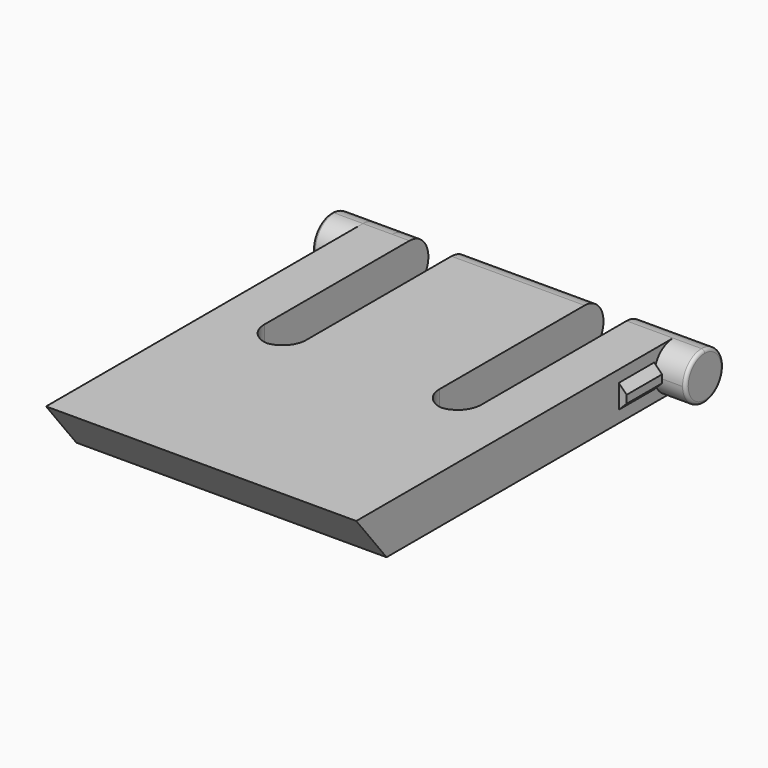
from build123d import *

# Parameters (mm, degrees)
F1_DEPTH      = 3
F3_DEPTH      = 2
F5_DEPTH      = 2
F6_DEPTH      = 0.5
F7_SIZE       = 0.49999
F8_DEPTH      = 0.5
F9_SIZE       = 0.49999
F10_DEPTH     = 19.66
F11_R         = 1.4999
F12_T3_DEPTH  = 3
F12_T6_DEPTH  = 3
F12_T9_DEPTH  = 3
F12_T12_DEPTH = 3
F12_T16_DEPTH = 15.94
F12_T19_DEPTH = 10.45
F12_T22_DEPTH = 15.94
F12_T25_DEPTH = 10.45
F14_T3_ANGLE  = 179.9999999988
F14_T6_ANGLE  = 90
F14_T9_ANGLE  = 90.0000000012


# Not quite as in the source:
# - a fillet or chamfer that OpenCascade refuses, or shapes differently, is made with other operations: its cross-section is extruded or revolved along the edge and cut away or added
# - two fillets or chamfers of one size are made in one step
# - a fillet or chamfer is up to 0.001 mm smaller than in the source, because OpenCascade refuses the exact size


with BuildPart() as f1:
    # F0 (on Top) → F1 (new body)
    with BuildSketch(Plane.XY):
        Polygon((-26.8430960169, 15.6478737652), (-29.7930960169, 15.6478737652), (-29.7930960169, -10.9521262348), (-10.1330960169, -10.9521262348), (-10.1330960169, 15.6478737652), (-13.0830960169, 15.6478737652), (-13.0830960169, 1.1478737652), (-15.7430960169, 1.1478737652), (-15.7430960169, 15.6478737652), (-24.1830960169, 15.6478737652), (-24.1830960169, 1.1478737652), (-26.8430960169, 1.1478737652), align=None)
    extrude(amount=F1_DEPTH)

    # F2 (on face) → F3 (join)
    with BuildSketch(Plane.YZ.offset(-10.1330960169)):
        with BuildLine():
            ThreePointArc((14.1478737652, 0), (15.208533937, 0.4393398282), (15.6478737652, 1.5))
            ThreePointArc((15.6478737652, 1.5), (15.208533937, 2.5606601718), (14.1478737652, 3))
            ThreePointArc((14.1478737652, 3), (13.0872135935, 2.5606601718), (12.6478737652, 1.5))
            ThreePointArc((12.6478737652, 1.5), (13.0872135935, 0.4393398282), (14.1478737652, 0))
        make_face()
    extrude(amount=F3_DEPTH)

    # F4 (on face) → F5 (join)
    with BuildSketch(Plane(origin=(-29.7930960169, 0, 0), x_dir=(0, -1, 0), z_dir=(-1, 0, 0))):
        with BuildLine():
            ThreePointArc((-14.1478737652, 0), (-13.0872135935, 0.4393398282), (-12.6478737652, 1.5))
            ThreePointArc((-12.6478737652, 1.5), (-13.0872135935, 2.5606601718), (-14.1478737652, 3))
            ThreePointArc((-14.1478737652, 3), (-15.2085339334, 2.5606601754), (-15.6478737652, 1.5000000103))
            ThreePointArc((-15.6478737652, 1.5000000103), (-15.2085339407, 0.4393398319), (-14.1478737652, 0))
        make_face()
    extrude(amount=F5_DEPTH)

    # F4 (on face) → F10 (cut, through all)
    with BuildSketch(Plane(origin=(-29.7930960169, 0, 0), x_dir=(0, -1, 0), z_dir=(-1, 0, 0))):
        Polygon((10.9521262348, 0), (10.9521262348, 3), (8.5521262348, 0), align=None)
    extrude(amount=-F10_DEPTH, mode=Mode.SUBTRACT)

    # F11 (radius 1.5 in the source; OpenCascade refuses exactly that, so slightly less here)
    f11_edges = [f1.edges().sort_by_distance(p)[0] for p in [
        (-28.318096, 15.647874, 3),
        (-28.318096, 15.647874, 0),
    ]]
    fillet(f11_edges, radius=F11_R)

    # F12: fillet of radius 1.5 on 8 edges, made by hand


with BuildPart() as f6:
    # F4 (on face) → F6 (new body)
    with BuildSketch(Plane(origin=(-29.7930960169, 0, 0), x_dir=(0, -1, 0), z_dir=(-1, 0, 0))):
        Polygon((-12.6478737652, 2.25), (-12.6478737652, 1.5), (-12.6478737652, 0.75), (-9.8478737652, 0.75), (-9.8478737652, 1.5), (-9.8478737652, 2.25), align=None)
    extrude(amount=F6_DEPTH)

    # F7 (size 0.5 in the source; OpenCascade refuses exactly that, so slightly less here)
    f7_edges = [f6.edges().sort_by_distance(p)[0] for p in [
        (-30.293096, 11.247874, 0.75),
        (-30.293096, 11.247874, 2.25),
    ]]
    chamfer(f7_edges, length=F7_SIZE)


with BuildPart() as f8:
    # F2 (on face) → F8 (new body)
    with BuildSketch(Plane.YZ.offset(-10.1330960169)):
        Polygon((12.6478737652, 0.75), (12.6478737652, 1.5), (12.6478737652, 2.25), (9.8478737652, 2.25), (9.8478737652, 0.75), align=None)
    extrude(amount=F8_DEPTH)

    # F9 (size 0.5 in the source; OpenCascade refuses exactly that, so slightly less here)
    f9_edges = [f8.edges().sort_by_distance(p)[0] for p in [
        (-9.633096, 11.247874, 2.25),
        (-9.633096, 11.247874, 0.75),
    ]]
    chamfer(f9_edges, length=F9_SIZE)


with BuildPart() as f12_tool1:
    # F12_s2 → F12_t3 (new body)
    with BuildSketch(Plane.XY):
        with BuildLine():
            ThreePointArc((-26.8430960169, 2.6478737652), (-26.4037561887, 1.5872135935), (-25.3430960169, 1.1478737652))
            Line((-25.3430960169, 1.1478737652), (-26.8430960169, 1.1478737652))
            Line((-26.8430960169, 1.1478737652), (-26.8430960169, 2.6478737652))
        make_face()
    extrude(amount=F12_T3_DEPTH)


with BuildPart() as f12_tool4:
    # F12_s5 → F12_t6 (new body)
    with BuildSketch(Plane.XY):
        with BuildLine():
            ThreePointArc((-25.6830960169, 1.1478737652), (-24.6224358452, 1.5872135935), (-24.1830960169, 2.6478737652))
            Line((-24.1830960169, 2.6478737652), (-24.1830960169, 1.1478737652))
            Line((-24.1830960169, 1.1478737652), (-25.6830960169, 1.1478737652))
        make_face()
    extrude(amount=F12_T6_DEPTH)


with BuildPart() as f12_tool7:
    # F12_s8 → F12_t9 (new body)
    with BuildSketch(Plane.XY):
        with BuildLine():
            ThreePointArc((-15.7430960169, 2.6478737652), (-15.3037561887, 1.5872135935), (-14.2430960169, 1.1478737652))
            Line((-14.2430960169, 1.1478737652), (-15.7430960169, 1.1478737652))
            Line((-15.7430960169, 1.1478737652), (-15.7430960169, 2.6478737652))
        make_face()
    extrude(amount=F12_T9_DEPTH)


with BuildPart() as f12_tool10:
    # F12_s11 → F12_t12 (new body)
    with BuildSketch(Plane.XY):
        with BuildLine():
            ThreePointArc((-13.0830960169, 2.6478737652), (-13.5224358452, 1.5872135935), (-14.5830960169, 1.1478737652))
            Line((-14.5830960169, 1.1478737652), (-13.0830960169, 1.1478737652))
            Line((-13.0830960169, 1.1478737652), (-13.0830960169, 2.6478737652))
        make_face()
    extrude(amount=F12_T12_DEPTH)


with BuildPart() as f1_1:
    add(f1.part)

    # F12_t13: union F12_tool1, F12_tool4, F12_tool7, F12_tool10
    add([f12_tool1.part, f12_tool4.part, f12_tool7.part, f12_tool10.part])


with BuildPart() as f12_tool14:
    # F12_s15 → F12_t16 (new body)
    with BuildSketch(Plane.YZ.offset(-11.9930960169)):
        with BuildLine():
            ThreePointArc((14.1478737652, 0), (15.208533937, 0.4393398282), (15.6478737652, 1.5))
            Line((15.6478737652, 1.5), (15.6478737652, 0))
            Line((15.6478737652, 0), (14.1478737652, 0))
        make_face()
    extrude(amount=-F12_T16_DEPTH)


with BuildPart() as f12_tool17:
    # F12_s18 → F12_t19 (new body)
    with BuildSketch(Plane.YZ.offset(-6.3830960169)):
        with BuildLine():
            ThreePointArc((14.1478737652, 0), (15.208533937, 0.4393398282), (15.6478737652, 1.5))
            Line((15.6478737652, 1.5), (15.6478737652, 0))
            Line((15.6478737652, 0), (14.1478737652, 0))
        make_face()
    extrude(amount=-F12_T19_DEPTH)


with BuildPart() as f12_tool20:
    # F12_s21 → F12_t22 (new body)
    with BuildSketch(Plane.YZ.offset(-11.9930960169)):
        with BuildLine():
            ThreePointArc((15.6478737652, 1.5), (15.208533937, 2.5606601718), (14.1478737652, 3))
            Line((14.1478737652, 3), (15.6478737652, 3))
            Line((15.6478737652, 3), (15.6478737652, 1.5))
        make_face()
    extrude(amount=-F12_T22_DEPTH)


with BuildPart() as f12_tool23:
    # F12_s24 → F12_t25 (new body)
    with BuildSketch(Plane.YZ.offset(-6.3830960169)):
        with BuildLine():
            ThreePointArc((15.6478737652, 1.5), (15.208533937, 2.5606601718), (14.1478737652, 3))
            Line((14.1478737652, 3), (15.6478737652, 3))
            Line((15.6478737652, 3), (15.6478737652, 1.5))
        make_face()
    extrude(amount=-F12_T25_DEPTH)


with BuildPart() as f1_2:
    add(f1_1.part)

    # F12_t26: cut F12_tool14, F12_tool17, F12_tool20, F12_tool23
    add([f12_tool14.part, f12_tool17.part, f12_tool20.part, f12_tool23.part], mode=Mode.SUBTRACT)

    # F14: fillet of radius 0.2 on 1 edges, made by hand


with BuildPart() as f14_tool1:
    # F14_s2 → F14_t3 (revolve)
    with BuildSketch(Plane.XZ.offset(-14.1478737652)):
        with BuildLine():
            ThreePointArc((-8.1330960169, 0.2), (-8.1916746607, 0.0585786438), (-8.3330960169, 0))
            Line((-8.3330960169, 0), (-8.1330960169, 0))
            Line((-8.1330960169, 0), (-8.1330960169, 0.2))
        make_face()
    revolve(axis=Axis((-8.1330960169, 14.1478737652, 1.5), (-1, 0, 0)), revolution_arc=F14_T3_ANGLE)


with BuildPart() as f14_tool4:
    # F14_s5 → F14_t6 (revolve)
    with BuildSketch(Plane.XY.offset(1.5)):
        with BuildLine():
            ThreePointArc((-8.3330960169, 15.6478737652), (-8.1916746607, 15.5892951215), (-8.1330960169, 15.4478737652))
            Line((-8.1330960169, 15.4478737652), (-8.1330960169, 15.6478737652))
            Line((-8.1330960169, 15.6478737652), (-8.3330960169, 15.6478737652))
        make_face()
    revolve(axis=Axis((-8.1330960169, 14.1478737652, 1.5), (-1, 0, 0)), revolution_arc=F14_T6_ANGLE)


with BuildPart() as f14_tool7:
    # F14_s8 → F14_t9 (revolve)
    with BuildSketch(Plane.XZ.offset(-14.1478737652)):
        with BuildLine():
            ThreePointArc((-8.3330960169, 3), (-8.1916746607, 2.9414213562), (-8.1330960169, 2.8))
            Line((-8.1330960169, 2.8), (-8.1330960169, 3))
            Line((-8.1330960169, 3), (-8.3330960169, 3))
        make_face()
    revolve(axis=Axis((-8.1330960169, 14.1478737652, 1.5), (-1, 0, 0)), revolution_arc=F14_T9_ANGLE)


with BuildPart() as f1_3:
    add(f1_2.part)

    # F14_t10: cut F14_tool1, F14_tool4, F14_tool7
    add([f14_tool1.part, f14_tool4.part, f14_tool7.part], mode=Mode.SUBTRACT)

    # F15: fillet of radius 0.2 on 1 edges, made by hand

    # F15_s1 → F15_t2 (revolve, cut)
    with BuildSketch(Plane.XY.offset(1.5)):
        with BuildLine():
            ThreePointArc((-31.5921303315, 15.6482737652), (-31.7345173732, 15.5892951215), (-31.7934960169, 15.4469080798))
            Line((-31.7934960169, 15.4469080798), (-31.8136325855, 15.4469080798))
            ThreePointArc((-31.8136325855, 15.4469080798), (-31.8132325855, 15.5473909225), (-31.8132325855, 15.6478737652))
            Line((-31.8132325855, 15.6478737652), (-31.7930960169, 15.6680103338))
            ThreePointArc((-31.7930960169, 15.6680103338), (-31.6926131742, 15.6680103338), (-31.5921303315, 15.6684103338))
            Line((-31.5921303315, 15.6684103338), (-31.5921303315, 15.6482737652))
        make_face()
    revolve(axis=Axis((-31.7930960169, 14.1478737652, 1.5), (1, 0, 0)), mode=Mode.SUBTRACT)


solid = Compound([f6.part, f8.part, f1_3.part])
